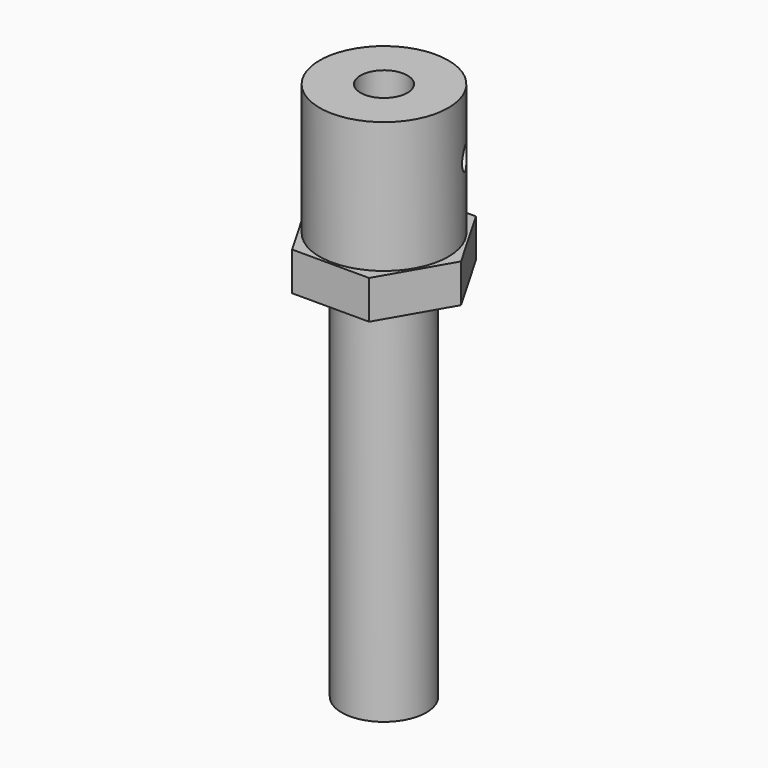
from build123d import *

# Parameters (mm, degrees)
F1_DEPTH = 4.99999
F2_R     = 8.34999981
F2_R_2   = 3.048
F3_DEPTH = 16.9999914
F4_R     = 1.4581169527
F5_DEPTH = 25.4
F6_R     = 5.5000017
F7_DEPTH = 47.999904
F9_DEPTH = 29.99994


# Not quite as in the source:
# - ends of sketch curves that miss each other by under 0.0002 mm in the source are joined


with BuildPart() as f1:
    # F0 (on Top) → F1 (new body)
    with BuildSketch(Plane.XY):
        Polygon((10.0000054, 0), (5.0000027, 8.6602587144), (-5.0000027, 8.6602587144), (-10.0000054, 0), (-5.0000027, -8.6602587144), (5.0000027, -8.6602587144), align=None)
    extrude(amount=F1_DEPTH)

    # F2 (on face) → F3 (join)
    with BuildSketch(Plane.XY.offset(4.99999)):
        Circle(F2_R)
        Circle(F2_R_2, mode=Mode.SUBTRACT)
    extrude(amount=F3_DEPTH)

    # F4 (on face) → F5 (cut)
    with BuildSketch(Plane(origin=(-7.50000405, -4.3301293572, 0), x_dir=(0.5, -0.8660254038, 0), z_dir=(-0.8660254038, -0.5, 0))):
        with Locations((0, 14.2499814)):
            Circle(F4_R)
    extrude(amount=-F5_DEPTH, mode=Mode.SUBTRACT)

    # F6 (on face) → F7 (join)
    with BuildSketch(Plane(origin=(0, 0, 0), x_dir=(1, 0, 0), z_dir=(0, 0, -1))):
        Circle(F6_R)
    extrude(amount=F7_DEPTH)

    # F8 (on face) → F9 (cut)
    with BuildSketch(Plane(origin=(0, 0, -47.999904), x_dir=(1, 0, 0), z_dir=(0, 0, -1))):
        with BuildLine():
            Line((2.5, -4.8989813941), (2.5, 0))
            ThreePointArc((2.5, 0), (0, 2.499995), (-2.499995, 0))
            Line((-2.499995, 0), (-2.5, -4.8989813941))
            ThreePointArc((-2.5, -4.8989813941), (0, -5.5000017), (2.5, -4.8989813941))
        make_face()
    extrude(amount=-F9_DEPTH, mode=Mode.SUBTRACT)


solid = f1.part
